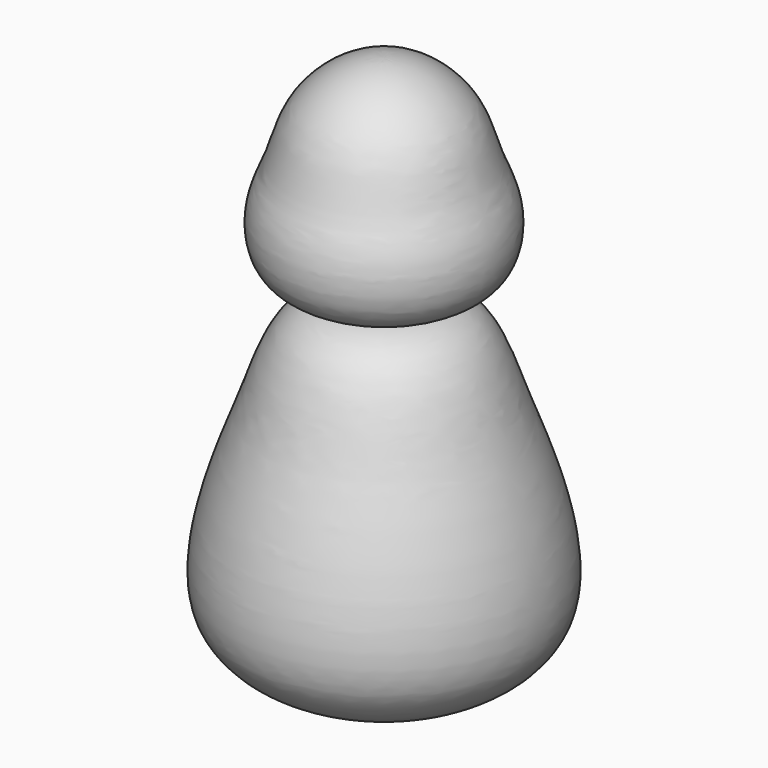
from build123d import *


# Not quite as in the source:
# - the dataset's text gives a spline's control points without its knots; the knots are read off the source's solid


with BuildPart() as f1:
    # F0 (on Front) → F1 (revolve)
    with BuildSketch(Plane.XZ):
        with BuildLine():
            Line((0.0828475478, 44.4510810842), (0, 47.625))
            Line((0, 47.625), (0, 0))
            Line((0, 0), (0.067537971, 3.1742815916))
            add(Edge.make_bspline(
                [(0.0828475478, 44.4510810842), (0.8259691177, 44.4704784921), (2.3129719527, 44.3754506266), (4.5277570417, 43.8632481161), (6.6875715628, 43.0153072301), (8.7417534692, 41.875510647), (10.6360876506, 40.4978573121), (12.0365888647, 39.2040697364), (13.0247440125, 38.1170616404), (13.6933377104, 37.2864551423), (14.2855495847, 36.4479482254), (14.9991836331, 35.2973566333), (15.7625324689, 33.805658), (16.5286089574, 31.9340383653), (17.0851525367, 30.3208456271), (17.5103993999, 29.0086661358), (17.8275229369, 28.0164165272), (18.1517283651, 27.0185764464), (18.4357007762, 26.1845144734), (18.6770989008, 25.516785706), (18.920459393, 24.8691283998), (19.22699954, 24.0896051963), (19.5898056302, 23.1979038166), (20.0572495505, 22.0575962077), (20.5945576958, 20.7058613351), (21.0385740922, 19.3982538763), (21.3269626385, 18.3381438994), (21.5075140524, 17.5242044354), (21.649423537, 16.6777672724), (21.7830575707, 15.4883830376), (21.8295470788, 13.9336212512), (21.6562151902, 12.0728895207), (21.2339168568, 10.3272991944), (20.6741544895, 9.0456955466), (20.1040740351, 8.1483871852), (19.6122439282, 7.5384923869), (19.0512031478, 6.9914303739), (18.362608675, 6.4588187943), (17.5516257551, 5.9536590548), (16.3106473808, 5.323769109), (14.4813496821, 4.6356651635), (11.9303638465, 3.995773159), (9.1207329887, 3.5436082772), (5.1538538848, 3.1745807045), (2.0648013383, 3.1317865856), (0.067537971, 3.1742815916)],
                knots=[0, 0, 0, 0, 0.03125, 0.0625, 0.09375, 0.125, 0.15625, 0.1874999999, 0.2031249999, 0.2187499999, 0.2343749999, 0.2499999999, 0.2812499999, 0.3124999999, 0.3437499999, 0.3593749999, 0.3749999999, 0.3906249999, 0.4062499999, 0.4140624999, 0.4218749999, 0.4374999999, 0.4531249999, 0.4687499999, 0.4999999998, 0.5312499998, 0.5468749998, 0.5624999998, 0.5781249998, 0.5937499998, 0.6249999998, 0.6562499998, 0.6874999998, 0.7187499998, 0.7343749998, 0.7499999998, 0.7656249998, 0.7812499998, 0.7968749998, 0.8124999998, 0.8437499997, 0.8749999997, 0.9062499997, 0.9374999997, 0.9999999997, 0.9999999997, 0.9999999997, 0.9999999997], degree=3))
        make_face()
        with BuildLine():
            add(Edge.make_bspline(
                [(0, 47.625), (6.6380382755, 47.7982700828), (18.1903953943, 40.2561558597), (21.0380439036, 26.7402773346), (25.7990612414, 18.0614575427), (24.2624997876, 1.4718581405), (8.0636420709, -0.1715670171), (0, 0)],
                knots=[0, 0, 0, 0, 0.2221316261, 0.4093656183, 0.5716098626, 0.7569257807, 1, 1, 1, 1], degree=3))
            Line((0, 47.625), (0.0828475478, 44.4510810842))
            add(Edge.make_bspline(
                [(0.0828475478, 44.4510810842), (0.8259691177, 44.4704784921), (2.3129719527, 44.3754506266), (4.5277570417, 43.8632481161), (6.6875715628, 43.0153072301), (8.7417534692, 41.875510647), (10.6360876506, 40.4978573121), (12.0365888647, 39.2040697364), (13.0247440125, 38.1170616404), (13.6933377104, 37.2864551423), (14.2855495847, 36.4479482254), (14.9991836331, 35.2973566333), (15.7625324689, 33.805658), (16.5286089574, 31.9340383653), (17.0851525367, 30.3208456271), (17.5103993999, 29.0086661358), (17.8275229369, 28.0164165272), (18.1517283651, 27.0185764464), (18.4357007762, 26.1845144734), (18.6770989008, 25.516785706), (18.920459393, 24.8691283998), (19.22699954, 24.0896051963), (19.5898056302, 23.1979038166), (20.0572495505, 22.0575962077), (20.5945576958, 20.7058613351), (21.0385740922, 19.3982538763), (21.3269626385, 18.3381438994), (21.5075140524, 17.5242044354), (21.649423537, 16.6777672724), (21.7830575707, 15.4883830376), (21.8295470788, 13.9336212512), (21.6562151902, 12.0728895207), (21.2339168568, 10.3272991944), (20.6741544895, 9.0456955466), (20.1040740351, 8.1483871852), (19.6122439282, 7.5384923869), (19.0512031478, 6.9914303739), (18.362608675, 6.4588187943), (17.5516257551, 5.9536590548), (16.3106473808, 5.323769109), (14.4813496821, 4.6356651635), (11.9303638465, 3.995773159), (9.1207329887, 3.5436082772), (5.1538538848, 3.1745807045), (2.0648013383, 3.1317865856), (0.067537971, 3.1742815916)],
                knots=[0, 0, 0, 0, 0.03125, 0.0625, 0.09375, 0.125, 0.15625, 0.1874999999, 0.2031249999, 0.2187499999, 0.2343749999, 0.2499999999, 0.2812499999, 0.3124999999, 0.3437499999, 0.3593749999, 0.3749999999, 0.3906249999, 0.4062499999, 0.4140624999, 0.4218749999, 0.4374999999, 0.4531249999, 0.4687499999, 0.4999999998, 0.5312499998, 0.5468749998, 0.5624999998, 0.5781249998, 0.5937499998, 0.6249999998, 0.6562499998, 0.6874999998, 0.7187499998, 0.7343749998, 0.7499999998, 0.7656249998, 0.7812499998, 0.7968749998, 0.8124999998, 0.8437499997, 0.8749999997, 0.9062499997, 0.9374999997, 0.9999999997, 0.9999999997, 0.9999999997, 0.9999999997], degree=3))
            Line((0.067537971, 3.1742815916), (0, 0))
        make_face()
    revolve(axis=Axis((0, 0, 23.8125), (0, 0, 1)))


with BuildPart() as f2:
    # F0 (on Front) → F2 (revolve)
    with BuildSketch(Plane.XZ):
        with BuildLine():
            Line((0.0828475478, 44.4510810842), (0, 47.625))
            Line((0, 47.625), (0, 0))
            Line((0, 0), (0.067537971, 3.1742815916))
            add(Edge.make_bspline(
                [(0.0828475478, 44.4510810842), (0.8259691177, 44.4704784921), (2.3129719527, 44.3754506266), (4.5277570417, 43.8632481161), (6.6875715628, 43.0153072301), (8.7417534692, 41.875510647), (10.6360876506, 40.4978573121), (12.0365888647, 39.2040697364), (13.0247440125, 38.1170616404), (13.6933377104, 37.2864551423), (14.2855495847, 36.4479482254), (14.9991836331, 35.2973566333), (15.7625324689, 33.805658), (16.5286089574, 31.9340383653), (17.0851525367, 30.3208456271), (17.5103993999, 29.0086661358), (17.8275229369, 28.0164165272), (18.1517283651, 27.0185764464), (18.4357007762, 26.1845144734), (18.6770989008, 25.516785706), (18.920459393, 24.8691283998), (19.22699954, 24.0896051963), (19.5898056302, 23.1979038166), (20.0572495505, 22.0575962077), (20.5945576958, 20.7058613351), (21.0385740922, 19.3982538763), (21.3269626385, 18.3381438994), (21.5075140524, 17.5242044354), (21.649423537, 16.6777672724), (21.7830575707, 15.4883830376), (21.8295470788, 13.9336212512), (21.6562151902, 12.0728895207), (21.2339168568, 10.3272991944), (20.6741544895, 9.0456955466), (20.1040740351, 8.1483871852), (19.6122439282, 7.5384923869), (19.0512031478, 6.9914303739), (18.362608675, 6.4588187943), (17.5516257551, 5.9536590548), (16.3106473808, 5.323769109), (14.4813496821, 4.6356651635), (11.9303638465, 3.995773159), (9.1207329887, 3.5436082772), (5.1538538848, 3.1745807045), (2.0648013383, 3.1317865856), (0.067537971, 3.1742815916)],
                knots=[0, 0, 0, 0, 0.03125, 0.0625, 0.09375, 0.125, 0.15625, 0.1874999999, 0.2031249999, 0.2187499999, 0.2343749999, 0.2499999999, 0.2812499999, 0.3124999999, 0.3437499999, 0.3593749999, 0.3749999999, 0.3906249999, 0.4062499999, 0.4140624999, 0.4218749999, 0.4374999999, 0.4531249999, 0.4687499999, 0.4999999998, 0.5312499998, 0.5468749998, 0.5624999998, 0.5781249998, 0.5937499998, 0.6249999998, 0.6562499998, 0.6874999998, 0.7187499998, 0.7343749998, 0.7499999998, 0.7656249998, 0.7812499998, 0.7968749998, 0.8124999998, 0.8437499997, 0.8749999997, 0.9062499997, 0.9374999997, 0.9999999997, 0.9999999997, 0.9999999997, 0.9999999997], degree=3))
        make_face()
    revolve(axis=Axis((0, 0, 23.8125), (0, 0, 1)))


with BuildPart() as f4:
    # F3 (on Front) → F4 (revolve)
    with BuildSketch(Plane.XZ):
        with BuildLine():
            add(Edge.make_bspline(
                [(0, 0), (10.0042552454, 0), (20.1534990403, -2.8370273331), (26.0091728923, -22.0413226573), (32.5212498809, -37.3573271092), (38.3022039612, -64.0989478859), (21.8354153186, -76.8949800842), (7.5690615594, -79.2950304351), (0, -79.375)],
                knots=[0, 0, 0, 0, 0.1660874353, 0.3211351087, 0.4804644216, 0.6663402882, 0.8243761042, 1, 1, 1, 1], degree=3))
            Line((0, 0), (0, -79.375))
        make_face()
    revolve(axis=Axis((0, 0, -39.6875), (0, 0, -1)))


solid = Compound([f1.part, f2.part, f4.part])
